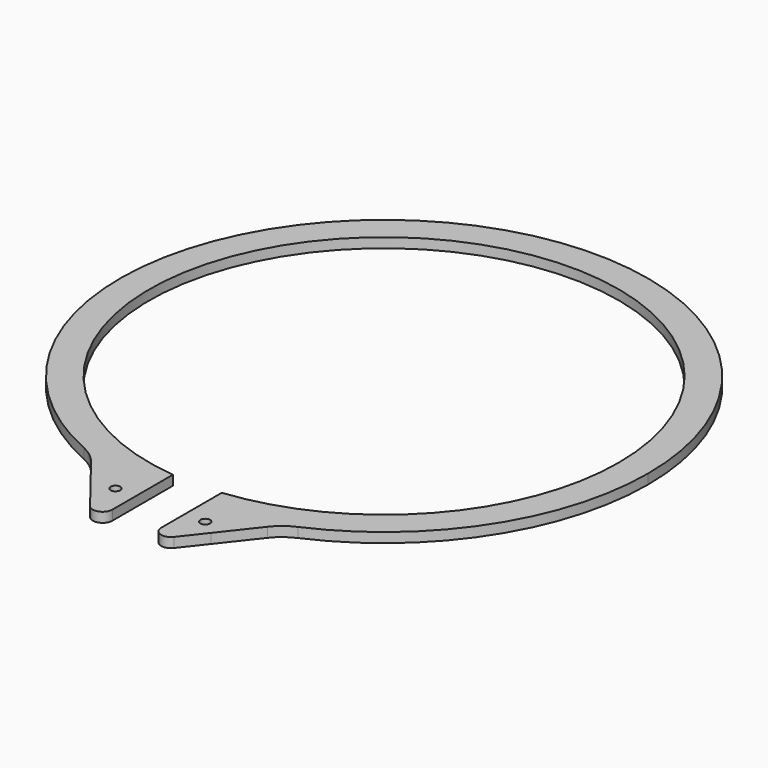
from build123d import *

# Parameters (mm, degrees)
F1_DEPTH = 1
F2_R     = 1
F3_R     = 1
F4_D     = 1
F4_DEPTH = 2
F4_TIP   = 0.3004303095
F5_R     = 5
F6_R     = 5


with BuildPart() as f1:
    # F0 (on Top) → F1 (new body)
    with BuildSketch(Plane.XY):
        with BuildLine():
            Line((-2.5, -34.5), (-2.5, -26.8840101175))
            ThreePointArc((-2.5, -26.8840101175), (-6.224328148, -26.2727565951), (-9.8270364159, -25.1481481481))
            Line((-9.8270364159, -25.1481481481), (-6.1635182079, -29.8240740741))
            Line((-6.1635182079, -29.8240740741), (-2.5, -34.5))
        make_face()
        with BuildLine():
            ThreePointArc((9.8270364159, -25.1481481481), (6.224328148, -26.2727565951), (2.5, -26.8840101175))
            Line((2.5, -26.8840101175), (2.5, -34.5))
            Line((2.5, -34.5), (6.1635182079, -29.8240740741))
            Line((6.1635182079, -29.8240740741), (9.8270364159, -25.1481481481))
        make_face()
        with BuildLine():
            Line((-2.5, -26.8840101175), (-2.5, -26.5288885241))
            Line((-2.5, -26.5288885241), (-9.8270364159, -25.1481481481))
            ThreePointArc((-9.8270364159, -25.1481481481), (-6.224328148, -26.2727565951), (-2.5, -26.8840101175))
        make_face()
        with BuildLine():
            Line((9.8270364159, -25.1481481481), (2.5, -26.5288885241))
            Line((2.5, -26.5288885241), (2.5, -26.8840101175))
            ThreePointArc((2.5, -26.8840101175), (6.224328148, -26.2727565951), (9.8270364159, -25.1481481481))
        make_face()
        with BuildLine():
            ThreePointArc((-2.5, -23.8694365246), (-16.0623784042, 17.8325545001), (24, 0))
            ThreePointArc((24, 0), (17.8325545001, -16.0623784042), (2.5, -23.8694365246))
            Line((2.5, -23.8694365246), (2.5, -26.5288885241))
            Line((2.5, -26.5288885241), (9.8270364159, -25.1481481481))
            ThreePointArc((9.8270364159, -25.1481481481), (22.2971969452, -15.2261291334), (27, 0))
            ThreePointArc((27, 0), (-15.2261291334, 22.2971969452), (-9.8270364159, -25.1481481481))
            Line((-9.8270364159, -25.1481481481), (-2.5, -26.5288885241))
            Line((-2.5, -26.5288885241), (-2.5, -23.8694365246))
        make_face()
    extrude(amount=F1_DEPTH)

    # F2
    f2_edges = [f1.edges().sort_by_distance(p)[0] for p in [
        (2.5, -34.5, 0.5),
    ]]
    fillet(f2_edges, radius=F2_R)

    # F3
    f3_edges = [f1.edges().sort_by_distance(p)[0] for p in [
        (-2.5, -34.5, 0.5),
    ]]
    fillet(f3_edges, radius=F3_R)

    # F4
    with Locations(Plane(origin=(0, 0, 0), x_dir=(1, 0, 0), z_dir=(0, 0, -1))):
        with Locations((-4.5891780847, 28.5906020734), (4.5891780847, 28.5906020734)):
            Hole(F4_D / 2, depth=F4_DEPTH)
            with Locations((0, 0, -(F4_DEPTH + F4_TIP / 2))):  # 118° drill point
                Cone(0, F4_D / 2, F4_TIP, mode=Mode.SUBTRACT)

    # F5
    f5_edges = [f1.edges().sort_by_distance(p)[0] for p in [
        (-9.827036, -25.148148, 0.5),
    ]]
    fillet(f5_edges, radius=F5_R)

    # F6
    f6_edges = [f1.edges().sort_by_distance(p)[0] for p in [
        (9.827036, -25.148148, 0.5),
    ]]
    fillet(f6_edges, radius=F6_R)


solid = f1.part
